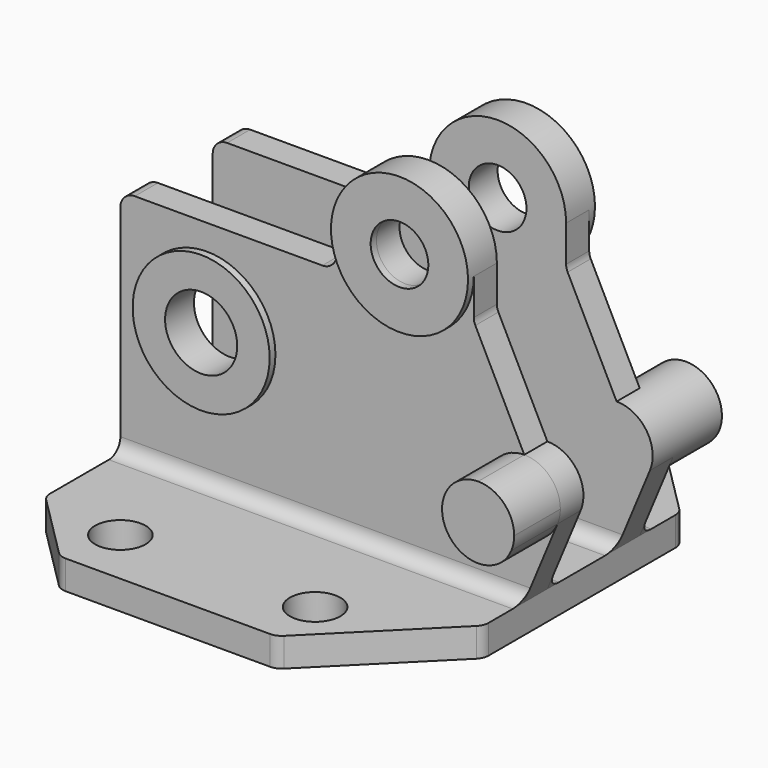
from build123d import *

# Parameters (mm, degrees)
F0_W           = 56
F0_H           = 66
F1_DEPTH       = 4
F3_D           = 7
F4_SIZE2       = 10
F4_SIZE        = 10
F5_SIZE2       = 16
F5_SIZE        = 16
F8_DEPTH       = 10
F8_DEPTH_BACK  = 10
F9_R           = 2
F11_R          = 5
F11_R_2        = 4
F12_DEPTH      = 20
F11_R_3        = 9.5
F13_DEPTH      = 1
F13_DEPTH_BACK = 21
F15_DEPTH      = 8
F15_DEPTH_BACK = 28
F10_W          = 12
F10_H          = 50
F16_DEPTH      = 61.001
F18_T4_DEPTH   = 56
F18_T9_DEPTH   = 61
F18_T15_DEPTH  = 56
F18_T20_DEPTH  = 61
F18_T26_DEPTH  = 56
F18_T31_DEPTH  = 61
F18_T37_DEPTH  = 56
F18_T42_DEPTH  = 61
F19_R          = 2


# Not quite as in the source:
# - a fillet or chamfer that OpenCascade refuses, or shapes differently, is made with other operations: its cross-section is extruded or revolved along the edge and cut away or added


with BuildPart() as f1:
    # F0 (on Top) → F1 (new body)
    with BuildSketch(Plane.XY):
        with Locations((28, 33)):
            Rectangle(F0_W, F0_H)
    extrude(amount=F1_DEPTH)

    # F3 (through all)
    with Locations(Plane.XY.offset(4)):
        with Locations((12, 58), (39, 58), (39, 8), (12, 8)):
            Hole(F3_D / 2)

    # F4
    f4_edges = [f1.edges().sort_by_distance(p)[0] for p in [
        (0, 66, 2),
        (0, 0, 2),
    ]]
    chamfer(f4_edges, length=F4_SIZE, length2=F4_SIZE2)

    # F5
    f5_edges = [f1.edges().sort_by_distance(p)[0] for p in [
        (56, 66, 2),
        (56, 0, 2),
    ]]
    chamfer(f5_edges, length=F5_SIZE, length2=F5_SIZE2)


with BuildPart() as f8:
    # F7 (on mid) → F8 (new body, two sides)
    with BuildSketch(Plane.XZ.offset(-33)) as f8_sk:
        with BuildLine():
            Line((0, 36), (0, 4))
            Line((0, 4), (56, 4))
            Line((56, 4), (60.6153846154, 15.0769230769))
            ThreePointArc((60.6153846154, 15.0769230769), (60.1602514717, 19.7735009811), (56, 22))
            Line((56, 22), (49, 36))
            Line((49, 36), (49, 41.5))
            ThreePointArc((49, 41.5), (39.5, 51), (30, 41.5))
            Line((30, 41.5), (30, 36))
            Line((30, 36), (0, 36))
        make_face()
    extrude(amount=-F8_DEPTH)
    extrude(f8_sk.sketch, amount=F8_DEPTH_BACK)

    # F9
    f9_edges = [f8.edges().sort_by_distance(p)[0] for p in [
        (30, 33, 36),
        (49, 33, 36),
        (0, 33, 36),
    ]]
    fillet(f9_edges, radius=F9_R)

    # F11 (on face) → F12 (cut, through all)
    with BuildSketch(Plane.XZ.offset(-23)):
        with Locations((12, 23)):
            Circle(F11_R)
        with Locations((39.5, 41.5)):
            Circle(F11_R_2)
    extrude(amount=-F12_DEPTH, mode=Mode.SUBTRACT)

    # F11 (on face) → F13 (join, two sides)
    with BuildSketch(Plane.XZ.offset(-23)) as f13_sk:
        with Locations((12, 23)):
            Circle(F11_R_3)
        with Locations((12, 23)):
            Circle(F11_R, mode=Mode.SUBTRACT)
        with BuildLine():
            ThreePointArc((30, 41.5), (39.5, 32), (49, 41.5))
            ThreePointArc((49, 41.5), (39.5, 51), (30, 41.5))
        make_face()
        with Locations((39.5, 41.5)):
            Circle(F11_R_2, mode=Mode.SUBTRACT)
    extrude(amount=F13_DEPTH)
    extrude(f13_sk.sketch, amount=-F13_DEPTH_BACK)

    # F14 (on face) → F15 (join, two sides)
    with BuildSketch(Plane.XZ.offset(-23)) as f15_sk:
        with BuildLine():
            ThreePointArc((60.6153846154, 15.0769230769), (60.9029033785, 16.0194193243), (61, 17))
            ThreePointArc((61, 17), (59.5355339059, 20.5355339059), (56, 22))
            ThreePointArc((56, 22), (51.8397485283, 14.2264990189), (60.6153846154, 15.0769230769))
        make_face()
    extrude(amount=F15_DEPTH)
    extrude(f15_sk.sketch, amount=-F15_DEPTH_BACK)

    # F10 (on face) → F16 (cut, through all)
    with BuildSketch(Plane(origin=(0, 0, 0), x_dir=(0, -1, 0), z_dir=(-1, 0, 0))):
        with Locations((-33, 29)):
            Rectangle(F10_W, F10_H)
    extrude(amount=-F16_DEPTH, mode=Mode.SUBTRACT)


with BuildPart() as f1_1:
    add(f1.part)

    # F17: union F8
    add(f8.part)

    # F18: fillet of radius 2 on 4 edges, made by hand


with BuildPart() as f18_tool2:
    # F18_s3 → F18_t4 (new body)
    with BuildSketch(Plane.YZ):
        with BuildLine():
            ThreePointArc((21, 4), (22.4142135624, 4.5857864376), (23, 6))
            Line((23, 6), (23, 4))
            Line((23, 4), (21, 4))
        make_face()
    extrude(amount=F18_T4_DEPTH)

    split(bisect_by=Plane(origin=(46.2958579882, 0, -19.2899408284), x_dir=(0, 1, 0), z_dir=(-0.9230769231, 0, 0.3846153846)), keep=Keep.TOP)


with BuildPart() as f1_2:
    add(f1_1.part)

    # F18_t1: union F18_tool2
    add(f18_tool2.part)


with BuildPart() as f18_tool7:
    # F18_s8 → F18_t9 (new body)
    with BuildSketch(Plane.YZ):
        with BuildLine():
            ThreePointArc((21, 4), (22.4142135624, 4.5857864376), (23, 6))
            Line((23, 6), (23, 4))
            Line((23, 4), (21, 4))
        make_face()
    extrude(amount=F18_T9_DEPTH)

    split(bisect_by=Plane.YZ.offset(56), keep=Keep.TOP)

    split(bisect_by=Plane(origin=(46.2958579882, 0, -19.2899408284), x_dir=(0, 1, 0), z_dir=(-0.9230769231, 0, 0.3846153846)), keep=Keep.TOP)


with BuildPart() as f1_3:
    add(f1_2.part)

    # F18_t6: union F18_tool7
    add(f18_tool7.part)


with BuildPart() as f18_tool13:
    # F18_s14 → F18_t15 (new body)
    with BuildSketch(Plane.YZ):
        with BuildLine():
            ThreePointArc((37, 4), (38.4142135624, 4.5857864376), (39, 6))
            Line((39, 6), (39, 4))
            Line((39, 4), (37, 4))
        make_face()
    extrude(amount=F18_T15_DEPTH)

    split(bisect_by=Plane(origin=(46.2958579882, 0, -19.2899408284), x_dir=(0, 1, 0), z_dir=(-0.9230769231, 0, 0.3846153846)), keep=Keep.TOP)


with BuildPart() as f1_4:
    add(f1_3.part)

    # F18_t12: union F18_tool13
    add(f18_tool13.part)


with BuildPart() as f18_tool18:
    # F18_s19 → F18_t20 (new body)
    with BuildSketch(Plane.YZ):
        with BuildLine():
            ThreePointArc((37, 4), (38.4142135624, 4.5857864376), (39, 6))
            Line((39, 6), (39, 4))
            Line((39, 4), (37, 4))
        make_face()
    extrude(amount=F18_T20_DEPTH)

    split(bisect_by=Plane.YZ.offset(56), keep=Keep.TOP)

    split(bisect_by=Plane(origin=(46.2958579882, 0, -19.2899408284), x_dir=(0, 1, 0), z_dir=(-0.9230769231, 0, 0.3846153846)), keep=Keep.TOP)


with BuildPart() as f1_5:
    add(f1_4.part)

    # F18_t17: union F18_tool18
    add(f18_tool18.part)


with BuildPart() as f18_tool24:
    # F18_s25 → F18_t26 (new body)
    with BuildSketch(Plane.YZ):
        with BuildLine():
            ThreePointArc((45, 4), (43.5857864376, 4.5857864376), (43, 6))
            Line((43, 6), (43, 4))
            Line((43, 4), (45, 4))
        make_face()
    extrude(amount=F18_T26_DEPTH)

    split(bisect_by=Plane(origin=(46.2958579882, 0, -19.2899408284), x_dir=(0, 1, 0), z_dir=(-0.9230769231, 0, 0.3846153846)), keep=Keep.TOP)


with BuildPart() as f1_6:
    add(f1_5.part)

    # F18_t23: union F18_tool24
    add(f18_tool24.part)


with BuildPart() as f18_tool29:
    # F18_s30 → F18_t31 (new body)
    with BuildSketch(Plane.YZ):
        with BuildLine():
            ThreePointArc((45, 4), (43.5857864376, 4.5857864376), (43, 6))
            Line((43, 6), (43, 4))
            Line((43, 4), (45, 4))
        make_face()
    extrude(amount=F18_T31_DEPTH)

    split(bisect_by=Plane.YZ.offset(56), keep=Keep.TOP)

    split(bisect_by=Plane(origin=(46.2958579882, 0, -19.2899408284), x_dir=(0, 1, 0), z_dir=(-0.9230769231, 0, 0.3846153846)), keep=Keep.TOP)


with BuildPart() as f1_7:
    add(f1_6.part)

    # F18_t28: union F18_tool29
    add(f18_tool29.part)


with BuildPart() as f18_tool35:
    # F18_s36 → F18_t37 (new body)
    with BuildSketch(Plane.YZ):
        with BuildLine():
            ThreePointArc((29, 4), (27.5857864376, 4.5857864376), (27, 6))
            Line((27, 6), (27, 4))
            Line((27, 4), (29, 4))
        make_face()
    extrude(amount=F18_T37_DEPTH)

    split(bisect_by=Plane(origin=(46.2958579882, 0, -19.2899408284), x_dir=(0, 1, 0), z_dir=(-0.9230769231, 0, 0.3846153846)), keep=Keep.TOP)


with BuildPart() as f1_8:
    add(f1_7.part)

    # F18_t34: union F18_tool35
    add(f18_tool35.part)


with BuildPart() as f18_tool40:
    # F18_s41 → F18_t42 (new body)
    with BuildSketch(Plane.YZ):
        with BuildLine():
            ThreePointArc((29, 4), (27.5857864376, 4.5857864376), (27, 6))
            Line((27, 6), (27, 4))
            Line((27, 4), (29, 4))
        make_face()
    extrude(amount=F18_T42_DEPTH)

    split(bisect_by=Plane.YZ.offset(56), keep=Keep.TOP)

    split(bisect_by=Plane(origin=(46.2958579882, 0, -19.2899408284), x_dir=(0, 1, 0), z_dir=(-0.9230769231, 0, 0.3846153846)), keep=Keep.TOP)


with BuildPart() as f1_9:
    add(f1_8.part)

    # F18_t39: union F18_tool40
    add(f18_tool40.part)

    # F19
    f19_edges = [f1_9.edges().sort_by_distance(p)[0] for p in [
        (40, 0, 2),
        (56, 16, 2),
        (10, 0, 2),
        (56, 50, 2),
        (40, 66, 2),
        (10, 66, 2),
        (0, 56, 2),
        (0, 10, 2),
    ]]
    fillet(f19_edges, radius=F19_R)


solid = f1_9.part
